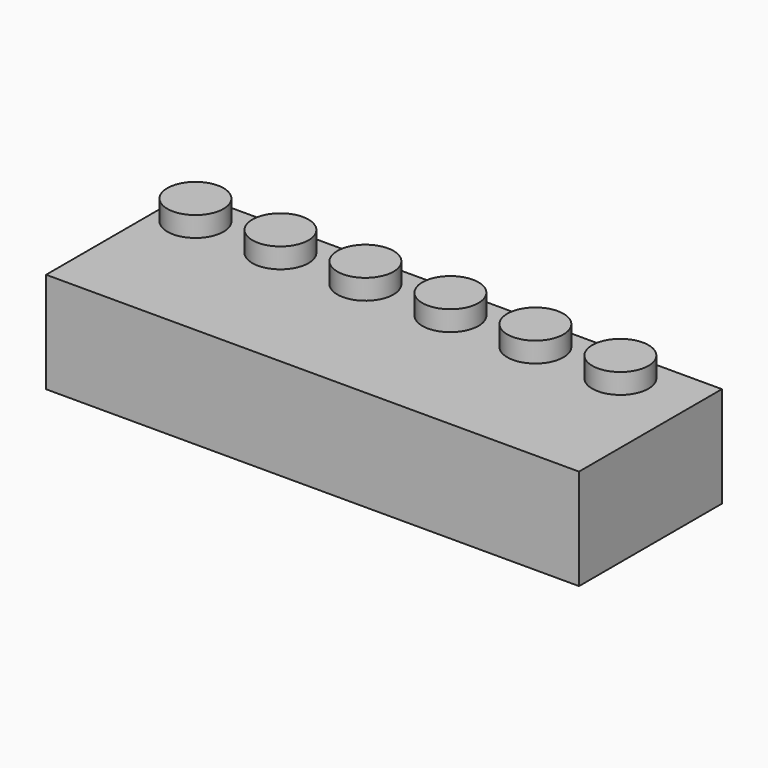
from build123d import *

# Parameters (mm, degrees)
F0_W     = 46.99
F0_H     = 15.748
F1_DEPTH = 8.89
F2_R     = 2.4765
F3_DEPTH = 1.778
F4_R     = 2.4765
F6_DEPTH = 1.778


# Not quite as in the source:
# - the program builds the solid bodies; features that only make, move or delete a surface that nothing else refers to are left out


with BuildPart() as f1:
    # F0 (on Top) → F1 (new body)
    with BuildSketch(Plane.XY):
        Rectangle(F0_W, F0_H)
    extrude(amount=F1_DEPTH)

    # F2 (on face) → F3 (join)
    with BuildSketch(Plane.XY.offset(8.89)):
        with Locations((-20.4343, 4.7625)):
            Circle(F2_R)
    extrude(amount=F3_DEPTH)

    # F4 (on face) → F6 (join)
    with BuildSketch(Plane.XY.offset(8.89)):
        with Locations((-12.9413, 4.7625)):
            Circle(F4_R)
        with Locations((-5.4483, 4.7625)):
            Circle(F4_R)
        with Locations((2.0447, 4.7625)):
            Circle(F4_R)
        with Locations((9.5377, 4.7625)):
            Circle(F4_R)
        with Locations((17.0307, 4.7625)):
            Circle(F4_R)
    extrude(amount=F6_DEPTH)


solid = f1.part
